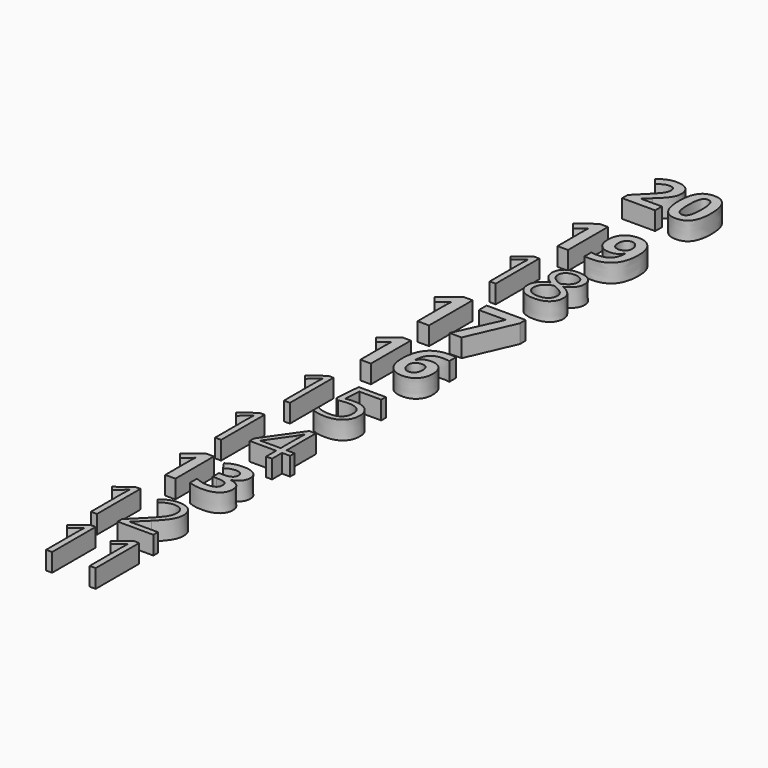
from build123d import *

# Parameters (mm, degrees)
F0_TEXT_SIZE   = 7.2287638889
F0_TEXT_SIZE_2 = 7.6388888889
F0_TEXT_SIZE_3 = 8.3333333333
F0_TEXT_SIZE_4 = 7.36775
F1_DEPTH       = 2


# Not quite as in the source:
# - Text() gives the source's letters only with a copy of the font that has no kerning and outlines rounded to 1/6400 em; it was checked with that copy


with BuildPart() as f1:
    # F0 (on Top) → F1 (new body)
    with BuildSketch(Plane.XY):
        with Locations((-16.8464660129, 66.6366429959)):
            Text('20', F0_TEXT_SIZE, font='Open Sans', font_style=FontStyle.BOLD, text_align=(TextAlign.LEFT, TextAlign.BOTTOM))
        with Locations((-17.3337941314, 56.2648866177)):
            Text('19', F0_TEXT_SIZE_2, font='Open Sans', font_style=FontStyle.BOLD, text_align=(TextAlign.LEFT, TextAlign.BOTTOM))
        with Locations((-18.0211856245, 47.5511574447)):
            Text('18', F0_TEXT_SIZE_3, font='Open Sans', text_align=(TextAlign.LEFT, TextAlign.BOTTOM))
        with Locations((-18.1722272911, 37.9606173635)):
            Text('17', F0_TEXT_SIZE_3, font='Open Sans', font_style=FontStyle.BOLD, text_align=(TextAlign.LEFT, TextAlign.BOTTOM))
        with Locations((-17.3564720828, 29.3530579507)):
            Text('16', F0_TEXT_SIZE_2, font='Open Sans', font_style=FontStyle.BOLD, text_align=(TextAlign.LEFT, TextAlign.BOTTOM))
        with Locations((-17.9730085411, 19.3627798259)):
            Text('15', F0_TEXT_SIZE_3, font='Open Sans', text_align=(TextAlign.LEFT, TextAlign.BOTTOM))
        with Locations((-18.2855085411, 10.3489266671)):
            Text('14', F0_TEXT_SIZE_3, font='Open Sans', text_align=(TextAlign.LEFT, TextAlign.BOTTOM))
        with Locations((-16.987315338, 2.3068100432)):
            Text('13', F0_TEXT_SIZE_4, font='Open Sans', font_style=FontStyle.BOLD, text_align=(TextAlign.LEFT, TextAlign.BOTTOM))
        with Locations((-18.0055606245, -6.9729444045)):
            Text('12', F0_TEXT_SIZE_3, font='Open Sans', text_align=(TextAlign.LEFT, TextAlign.BOTTOM))
        with Locations((-16.5967064578, -14.8638428822)):
            Text('11', F0_TEXT_SIZE_3, font='Open Sans', text_align=(TextAlign.LEFT, TextAlign.BOTTOM))
    extrude(amount=F1_DEPTH)


solid = f1.part
